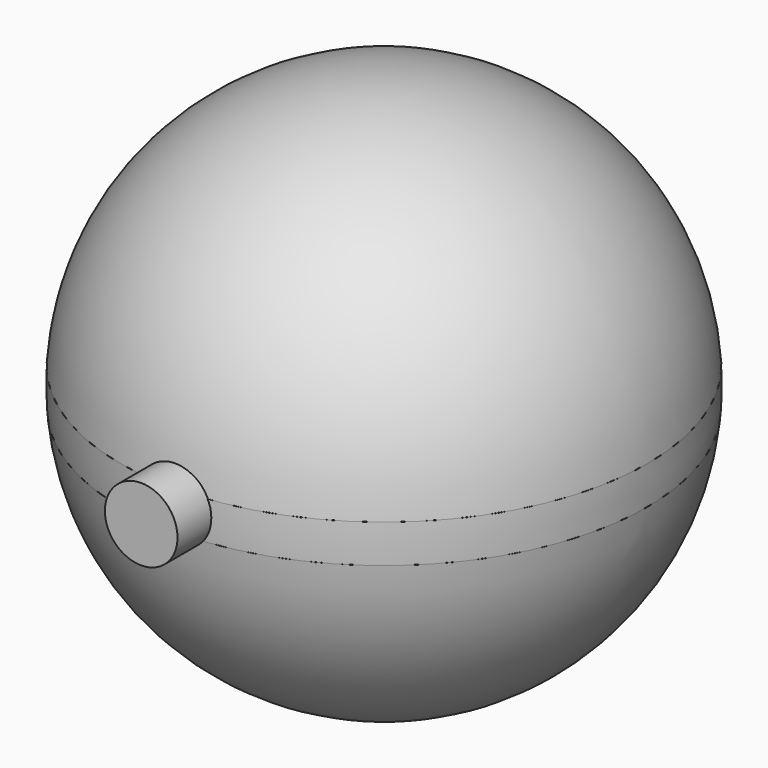
from build123d import *

# Parameters (mm, degrees)
F5_R     = 6.9898511366
F6_DEPTH = 58.42


# Not quite as in the source:
# - a feature names something its author has since deleted; it is built from what else it names


with BuildPart() as f1:
    # F0 (on Front) → F1 (revolve)
    with BuildSketch(Plane.XZ):
        with BuildLine():
            Line((0, 2.9950267635), (50.7116339185, 2.9950267635))
            ThreePointArc((50.7116339185, 2.9950267635), (34.8460373673, 36.9647626774), (0, 50.8))
            Line((0, 50.8), (0, 2.9950267635))
        make_face()
    revolve(axis=Axis((0, 0, -2.1393038332), (0, 0, -1)))


with BuildPart() as f1b:
    # F0 (on Front) → F1, piece 2 (revolve)
    with BuildSketch(Plane.XZ):
        with BuildLine():
            ThreePointArc((0, -50.8), (34.3223070251, -37.4515585854), (50.6072398558, -4.4212299399))
            Line((50.6072398558, -4.4212299399), (0, -4.4212299399))
            Line((0, -4.4212299399), (0, -50.8))
        make_face()
    revolve(axis=Axis((0, 0, -2.1393038332), (0, 0, -1)))


with BuildPart() as f3:
    # F0 (on Front) → F3 (revolve)
    with BuildSketch(Plane.XZ):
        with BuildLine():
            Line((0, -4.4212299399), (0, 2.9950267635))
            Line((0, 2.9950267635), (-50.7116339185, 2.9950267635))
            ThreePointArc((-50.7116339185, 2.9950267635), (-50.7949678767, -0.7150093742), (-50.6072398558, -4.4212299399))
            Line((-50.6072398558, -4.4212299399), (0, -4.4212299399))
        make_face()
    revolve(axis=Axis((0, 0, -2.5671664625), (0, 0, -1)))


with BuildPart() as f6:
    # F5 (on Front) → F6 (new body)
    with BuildSketch(Plane.XZ):
        Circle(F5_R)
    extrude(amount=F6_DEPTH)


solid = Compound([f1.part, f1b.part, f3.part, f6.part])
